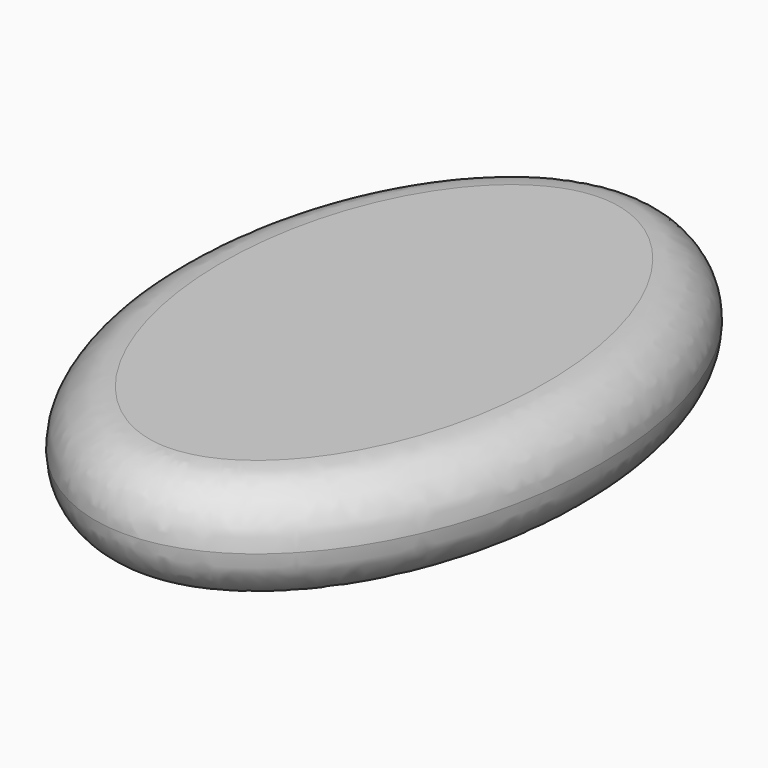
from build123d import *

# Parameters (mm, degrees)
F1_DEPTH = 6.35
F2_R     = 3.17499


# Not quite as in the source:
# - a fillet or chamfer is up to 0.001 mm smaller than in the source, because OpenCascade refuses the exact size


with BuildPart() as f1:
    # F0 (on Top) → F1 (new body)
    with BuildSketch(Plane.XY):
        with BuildLine():
            add(Edge.make_bspline(
                [(0, -19.05), (21.9970452561, -19.05), (10.9985226281, 9.525), (0, 38.1), (-10.9985226281, 9.525), (-21.9970452561, -19.05), (0, -19.05)],
                knots=[0, 0, 0, 2.0943951024, 2.0943951024, 4.1887902048, 4.1887902048, 6.2831853072, 6.2831853072, 6.2831853072], degree=2, weights=[1, 0.5, 1, 0.5, 1, 0.5, 1]))
        make_face()
    extrude(amount=F1_DEPTH)

    # F2 (radius 3.175 in the source; OpenCascade refuses exactly that, so slightly less here)
    f2_edges = [f1.edges().sort_by_distance(p)[0] for p in [
        (0, 19.05, 6.35),
        (0, 19.05, 0),
    ]]
    fillet(f2_edges, radius=F2_R)


solid = f1.part
